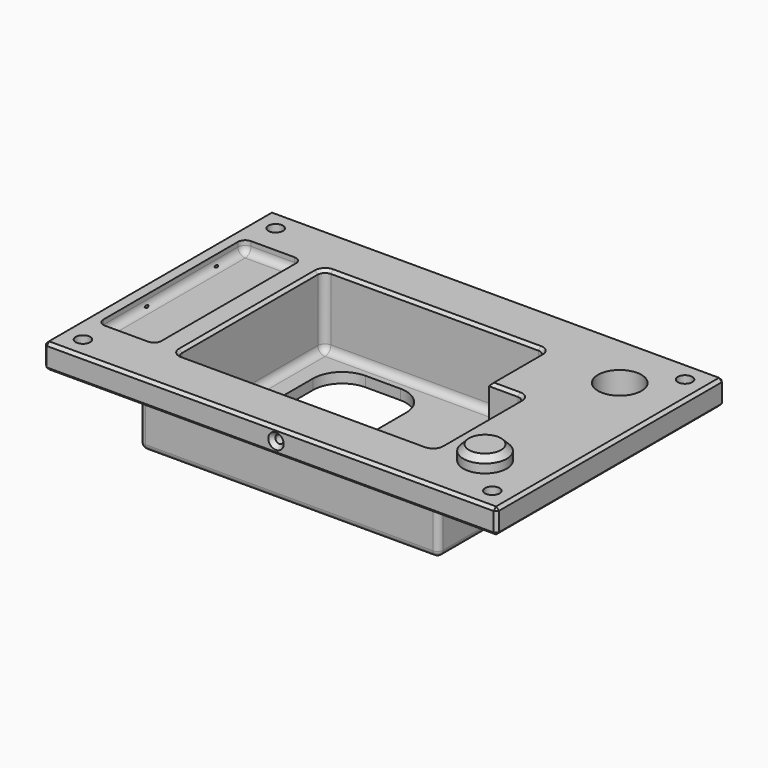
from build123d import *

# Parameters (mm, degrees)
F0_W            = 396.24
F0_H            = 248.92
F1_DEPTH        = 21.59
F3_DEPTH        = 50.8
F5_DEPTH        = 63.5
F6_R            = 6.35
F7_R            = 5.08
F8_W            = 81.28
F8_H            = 137.16
F9_DEPTH        = 72.391
F10_W           = 50.8
F10_H           = 160.02
F11_DEPTH       = 10.414
F12_R           = 6.35
F13_R           = 19.05
F14_DEPTH       = 12.7
F15_SIZE        = 5.08
F17_D           = 7.1374
F17_DEPTH       = 127
F17_CSINK_D     = 13.4874
F17_CSINK_ANGLE = 82
F17_TIP         = 2.1442912911
F18_R           = 5.08
F20_D           = 12.7
F20_CBORE_D     = 22.225
F20_CBORE_DEPTH = 12.7
F21_R           = 19.05
F22_DEPTH       = 72.391
F24_SIZE        = 2.54
F25_R           = 25.4
F26_D           = 8.7376
F26_DEPTH       = 12.7
F26_TIP         = 2.6250398724


with BuildPart() as f1:
    # F0 (on Top) → F1 (new body)
    with BuildSketch(Plane.XY):
        Rectangle(F0_W, F0_H)
    extrude(amount=-F1_DEPTH)

    # F2 (on face) → F3 (join)
    with BuildSketch(Plane(origin=(0, 0, -21.59), x_dir=(1, 0, 0), z_dir=(0, 0, -1))):
        Polygon((127, 99.06), (-134.62, 99.06), (-134.62, -97.79), (95.25, -97.79), (95.25, -35.56), (127, -35.56), align=None)
    extrude(amount=F3_DEPTH)

    # F4 (on face) → F5 (cut)
    with BuildSketch(Plane.XY):
        Polygon((-116.84, -81.28), (109.22, -81.28), (109.22, 17.78), (77.47, 17.78), (77.47, 80.01), (-116.84, 80.01), align=None)
    extrude(amount=-F5_DEPTH, mode=Mode.SUBTRACT)

    # F6
    f6_edges = [f1.edges().sort_by_distance(p)[0] for p in [
        (-3.81, -81.28, -63.5),
        (109.22, -31.75, -63.5),
        (93.345, 17.78, -63.5),
        (77.47, 48.895, -63.5),
        (-19.685, 80.01, -63.5),
        (-116.84, -0.635, -63.5),
        (109.22, -81.28, -31.75),
        (-116.84, -81.28, -31.75),
        (-116.84, 80.01, -31.75),
        (109.22, 17.78, -31.75),
        (77.47, 80.01, -31.75),
    ]]
    fillet(f6_edges, radius=F6_R)

    # F7
    f7_edges = [f1.edges().sort_by_distance(p)[0] for p in [
        (95.25, 35.56, -46.99),
    ]]
    fillet(f7_edges, radius=F7_R)

    # F8 (on face) → F9 (cut, through all)
    with BuildSketch(Plane(origin=(0, 0, -72.39), x_dir=(1, 0, 0), z_dir=(0, 0, -1))):
        with Locations((-55.88, 0)):
            Rectangle(F8_W, F8_H)
    extrude(amount=-F9_DEPTH, mode=Mode.SUBTRACT)

    # F10 (on face) → F11 (cut)
    with BuildSketch(Plane.XY):
        with Locations((-161.29, 0)):
            Rectangle(F10_W, F10_H)
    extrude(amount=-F11_DEPTH, mode=Mode.SUBTRACT)

    # F12
    f12_edges = [f1.edges().sort_by_distance(p)[0] for p in [
        (-135.89, 0, -10.414),
        (-161.29, 80.01, -10.414),
        (-186.69, 0, -10.414),
        (-161.29, -80.01, -10.414),
        (-186.69, 80.01, -5.207),
        (-135.89, 80.01, -5.207),
        (-135.89, -80.01, -5.207),
        (-186.69, -80.01, -5.207),
    ]]
    fillet(f12_edges, radius=F12_R)

    # F13 (on face) → F14 (join)
    with BuildSketch(Plane.XY):
        with Locations((147.32, -73.66)):
            Circle(F13_R)
    extrude(amount=F14_DEPTH)

    # F15
    f15_edges = [f1.edges().sort_by_distance(p)[0] for p in [
        (128.27, -73.66, 12.7),
    ]]
    chamfer(f15_edges, length=F15_SIZE)

    # F17
    with Locations(Plane.XZ.offset(124.46)):
        with Locations((5.08, -10.668)):
            CounterSinkHole(F17_D / 2, F17_CSINK_D / 2, depth=F17_DEPTH, counter_sink_angle=F17_CSINK_ANGLE)
            with Locations((0, 0, -(F17_DEPTH + F17_TIP / 2))):  # 118° drill point
                Cone(0, F17_D / 2, F17_TIP, mode=Mode.SUBTRACT)

    # F18
    f18_edges = [f1.edges().sort_by_distance(p)[0] for p in [
        (-3.81, -99.06, -72.39),
        (-134.62, -99.06, -46.99),
        (-134.62, -0.635, -72.39),
        (127, -31.75, -72.39),
        (127, -99.06, -46.99),
        (127, 35.56, -46.99),
        (113.665, 35.56, -72.39),
        (95.25, 97.79, -46.99),
        (-19.685, 97.79, -72.39),
        (-134.62, 97.79, -46.99),
    ]]
    fillet(f18_edges, radius=F18_R)

    # F20 (through all)
    with Locations(Plane(origin=(0, 0, -21.59), x_dir=(1, 0, 0), z_dir=(0, 0, -1))):
        with Locations((-179.07, 105.41), (179.07, 105.41), (179.07, -105.41), (-179.07, -105.41)):
            CounterBoreHole(F20_D / 2, F20_CBORE_D / 2, F20_CBORE_DEPTH)

    # F21 (on face) → F22 (cut, through all)
    with BuildSketch(Plane.XY):
        with Locations((147.32, 73.66)):
            Circle(F21_R)
    extrude(amount=-F22_DEPTH, mode=Mode.SUBTRACT)

    # F24
    f24_edges = [f1.edges().sort_by_distance(p)[0] for p in [
        (198.12, 124.46, -10.795),
        (-198.12, 124.46, -10.795),
        (0, 124.46, 0),
        (0, 124.46, -21.59),
        (198.12, -124.46, -10.795),
        (198.12, 0, 0),
        (198.12, 0, -21.59),
        (-198.12, -124.46, -10.795),
        (-198.12, 0, 0),
        (-198.12, 0, -21.59),
        (90.17, 17.78, 0),
        (0, -124.46, -21.59),
        (0, -124.46, 0),
    ]]
    chamfer(f24_edges, length=F24_SIZE)

    # F25
    f25_edges = [f1.edges().sort_by_distance(p)[0] for p in [
        (-15.24, -68.58, -67.945),
        (-15.24, 68.58, -67.945),
        (-96.52, 68.58, -67.945),
        (-96.52, -68.58, -67.945),
    ]]
    fillet(f25_edges, radius=F25_R)

    # F26
    with Locations(Plane(origin=(-198.12, 0, 0), x_dir=(0, -1, 0), z_dir=(-1, 0, 0))):
        with Locations((-48.26, -11.7549253628), (27.94, -11.7549253628), (73.66, -11.7549253628), (-99.06, -11.7549253628)):
            Hole(F26_D / 2, depth=F26_DEPTH)
            with Locations((0, 0, -(F26_DEPTH + F26_TIP / 2))):  # 118° drill point
                Cone(0, F26_D / 2, F26_TIP, mode=Mode.SUBTRACT)


solid = f1.part
